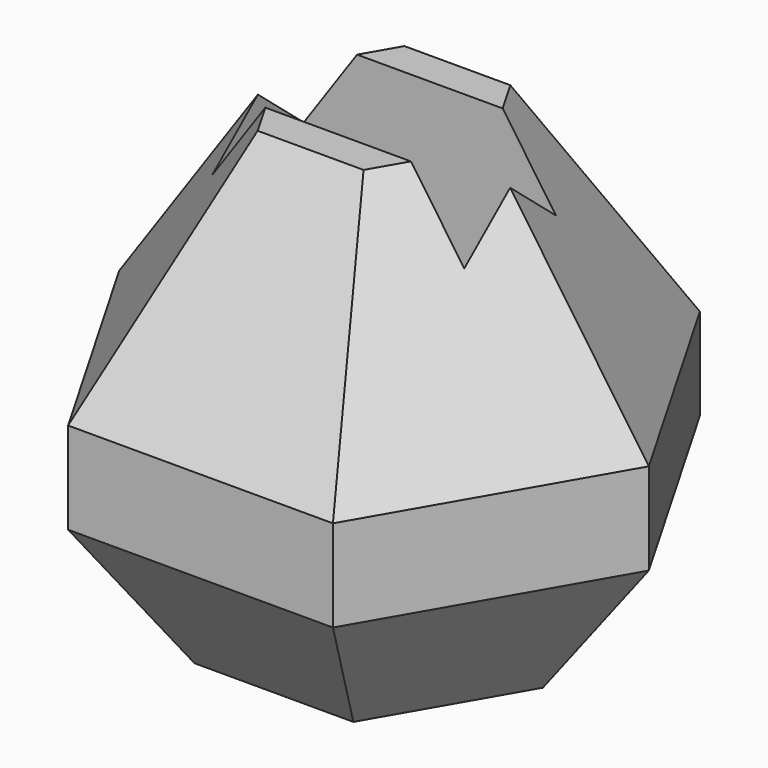
from build123d import *

# Parameters (mm, degrees)
F0_W        = 5.5
F0_H        = 2.5
F1_DEPTH    = 10
F2_T1_DEPTH = 21.2763058351
F2_T3_DEPTH = 21.2763058351
F2_T5_DEPTH = 21.2763058351
F2_T7_DEPTH = 21.2763058351
F2_T9_DEPTH = 21.2763058351
F3_T1_DEPTH = 31.6361136638
F3_T3_DEPTH = 31.6361136638
F3_T5_DEPTH = 31.6361136638
F3_T7_DEPTH = 31.6361136638
F3_T9_DEPTH = 31.6361136638
F4_DEPTH    = 5


# Not quite as in the source:
# - a fillet or chamfer that OpenCascade refuses, or shapes differently, is made with other operations: its cross-section is extruded or revolved along the edge and cut away or added


with BuildPart() as f1:
    # F0 (on Top) → F1 (new body)
    with BuildSketch(Plane.XY):
        Polygon((2.8867513459, 5), (-2.8867513459, 5), (-5.7735026919, 0), (-2.8867513459, -5), (2.8867513459, -5), (5.7735026919, 0), align=None)
        Rectangle(F0_W, F0_H, mode=Mode.SUBTRACT)
    extrude(amount=F1_DEPTH)

    # F2: chamfer of 2 x 3 on 6 edges, made by hand

    # F2_s2 → F2_t1 (cut)
    with BuildSketch(Plane.YZ.offset(-10.6381529176)):
        Polygon((5, 3), (3, 0), (5, 0), align=None)
        Polygon((-5, 3), (-3, 0), (-5, 0), align=None)
    extrude(amount=F2_T1_DEPTH, mode=Mode.SUBTRACT)

    # F2_s4 → F2_t3 (cut)
    with BuildSketch(Plane(origin=(5.3190764588, -9.212910676, 0), x_dir=(0, 0, 1), z_dir=(-0.5, 0.8660254038, 0))):
        Polygon((3, 5), (0, 3), (0, 5), align=None)
    extrude(amount=F2_T3_DEPTH, mode=Mode.SUBTRACT)

    # F2_s6 → F2_t5 (cut)
    with BuildSketch(Plane(origin=(5.3190764588, 9.212910676, 0), x_dir=(0, 0, 1), z_dir=(-0.5, -0.8660254038, 0))):
        Polygon((3, 5), (0, 3), (0, 5), align=None)
    extrude(amount=F2_T5_DEPTH, mode=Mode.SUBTRACT)

    # F2_s8 → F2_t7 (cut)
    with BuildSketch(Plane(origin=(-5.3190764588, 9.212910676, 0), x_dir=(0, 0, 1), z_dir=(0.5, -0.8660254038, 0))):
        Polygon((3, 5), (0, 3), (0, 5), align=None)
    extrude(amount=F2_T7_DEPTH, mode=Mode.SUBTRACT)

    # F2_s10 → F2_t9 (cut)
    with BuildSketch(Plane(origin=(-5.3190764588, -9.212910676, 0), x_dir=(0, 0, 1), z_dir=(0.5, 0.8660254038, 0))):
        Polygon((3, 5), (0, 3), (0, 5), align=None)
    extrude(amount=F2_T9_DEPTH, mode=Mode.SUBTRACT)

    # F3: chamfer of 5 x 3 on 6 edges, made by hand

    # F3_s2 → F3_t1 (cut)
    with BuildSketch(Plane(origin=(7.909028416, -13.6988390549, 0), x_dir=(0, 0, 1), z_dir=(-0.5, 0.8660254038, 0))):
        Polygon((5, 5), (10, 2), (10, 5), align=None)
    extrude(amount=F3_T1_DEPTH, mode=Mode.SUBTRACT)

    # F3_s4 → F3_t3 (cut)
    with BuildSketch(Plane.YZ.offset(-15.8180568319)):
        Polygon((5, 5), (2, 10), (5, 10), align=None)
        Polygon((-2, 10), (-5, 5), (-5, 10), align=None)
    extrude(amount=F3_T3_DEPTH, mode=Mode.SUBTRACT)

    # F3_s6 → F3_t5 (cut)
    with BuildSketch(Plane(origin=(7.909028416, 13.6988390549, 0), x_dir=(0, 0, 1), z_dir=(-0.5, -0.8660254038, 0))):
        Polygon((10, 2), (5, 5), (10, 5), align=None)
    extrude(amount=F3_T5_DEPTH, mode=Mode.SUBTRACT)

    # F3_s8 → F3_t7 (cut)
    with BuildSketch(Plane(origin=(-7.909028416, 13.6988390549, 0), x_dir=(0, 0, 1), z_dir=(0.5, -0.8660254038, 0))):
        Polygon((10, 2), (5, 5), (10, 5), align=None)
    extrude(amount=F3_T7_DEPTH, mode=Mode.SUBTRACT)

    # F3_s10 → F3_t9 (cut)
    with BuildSketch(Plane(origin=(-7.909028416, -13.6988390549, 0), x_dir=(0, 0, 1), z_dir=(0.5, 0.8660254038, 0))):
        Polygon((10, 2), (5, 5), (10, 5), align=None)
    extrude(amount=F3_T9_DEPTH, mode=Mode.SUBTRACT)

    # F0 (on Top) → F4 (join)
    with BuildSketch(Plane.XY):
        Rectangle(F0_W, F0_H)
    extrude(amount=F4_DEPTH)


solid = f1.part
